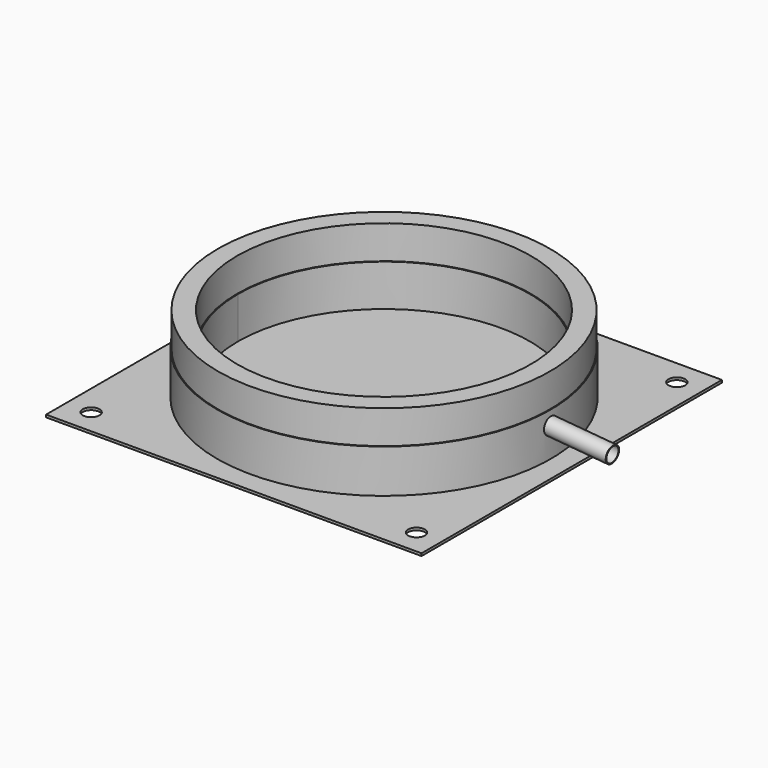
from build123d import *
from build123d import SkipClean  # not in build123d's __all__

# Parameters (mm, degrees)
F0_W     = 10
F0_H     = 3
F2_W     = 450
F2_H     = 450
F2_R     = 10
F3_DEPTH = 3
F6_R     = 9
F7_DEPTH = 120
F8_R     = 175
F9_DEPTH = 200


with BuildPart() as f1:
    # F0 (on Front) → F1 (revolve)
    with BuildSketch(Plane.XZ):
        Polygon((-200, 5), (-175, 5), (-175, 55), (-176, 55), (-176, 95), (-199, 95), (-199, 55), (-200, 55), align=None)
        Polygon((-10, 5), (-175, 5), (-200, 5), (-200, 2), (-10, 2), align=None)
        with Locations((-5, 3.5)):
            Rectangle(F0_W, F0_H)
    revolve(axis=Axis((0, 0, 187.9212413023), (0, 0, -1)))

    # F2 (on Top) → F3 (join)
    with BuildSketch(Plane.XY):
        Rectangle(F2_W, F2_H)
        with Locations((-195, -195)):
            Circle(F2_R, mode=Mode.SUBTRACT)
        with Locations((195, -195)):
            Circle(F2_R, mode=Mode.SUBTRACT)
        with Locations((-195, 195)):
            Circle(F2_R, mode=Mode.SUBTRACT)
        with Locations((195, 195)):
            Circle(F2_R, mode=Mode.SUBTRACT)
    extrude(amount=F3_DEPTH)

    # F4 (on Front) → F5 (revolve)
    with BuildSketch(Plane.XZ):
        Polygon((274.6194698092, 41.5098406888), (175, 50.2254149636), (174.9128442573, 49.2292202655), (274.5323140664, 40.5136459907), align=None)
    revolve(axis=Axis((287.7442754949, 0, 30.3233706049), (0.9961946981, 0, -0.0871557427)))

    # F6 (on face) → F7 (cut)
    with BuildSketch(Plane(origin=(268.9293723072, 0, -23.528271366), x_dir=(0, 1, 0), z_dir=(0.9961946981, 0, -0.0871557427))):
        with Locations((0, 55.286547077)):
            Circle(F6_R)
    extrude(amount=-F7_DEPTH, mode=Mode.SUBTRACT)

    # F8 (on face) → F9 (cut)
    with BuildSketch(Plane.XY.offset(5)):
        Circle(F8_R)
    with SkipClean():  # cleaning this boolean's faces spoils the solid; the shape is the same uncleaned
        extrude(amount=F9_DEPTH, mode=Mode.SUBTRACT)


solid = f1.part
